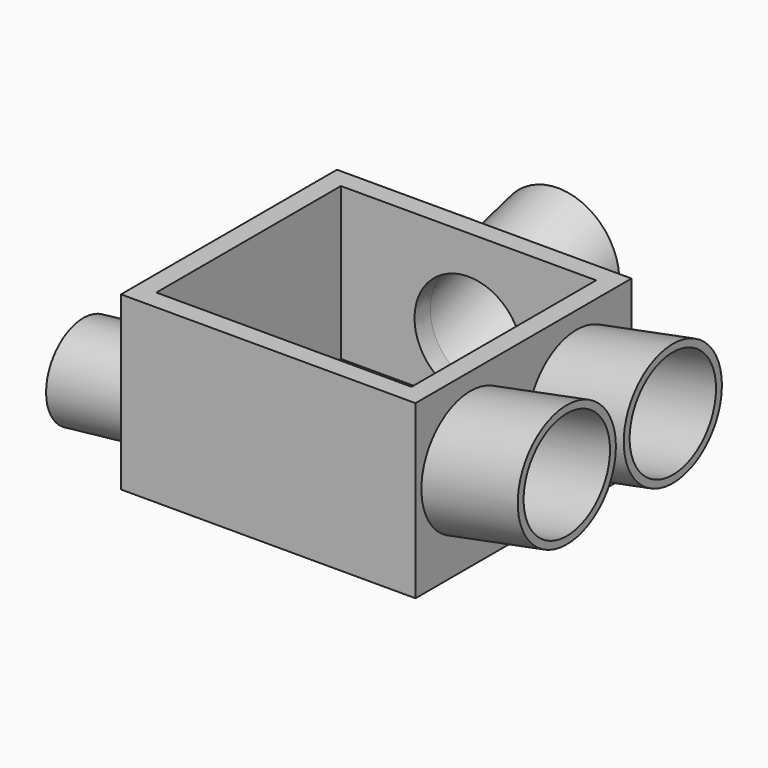
from build123d import *

# Parameters (mm, degrees)
F0_W      = 60
F0_H      = 55
F1_DEPTH  = 35
F2_T      = -4
F3_R      = 9.5
F3_R_2    = 8
F6_R      = 8
F7_DEPTH  = 4
F8_R      = 12.5
F8_R_2    = 11
F11_R     = 11
F12_DEPTH = 4
F13_R     = 12.5
F13_R_2   = 11
F16_DEPTH = 4


with BuildPart() as f1:
    # F0 (on Top) → F1 (new body)
    with BuildSketch(Plane.XY):
        Rectangle(F0_W, F0_H)
    extrude(amount=F1_DEPTH)

    # F2
    f2_openings = [f1.faces().sort_by_distance(p)[0] for p in [
        (0, 0, 35),
    ]]
    offset(amount=F2_T, openings=f2_openings)

    # F5: sweep along a path in F4
    with BuildLine(Plane.XZ) as f5_path:
        Line((-30, 12.8732416779), (-49.8803923108, 10.6892083519))
    # F3 (on face) → F5 (sweep)
    with BuildSketch(Plane(origin=(-30, 0, 0), x_dir=(0, -1, 0), z_dir=(-1, 0, 0))):
        with Locations((12.2240986817, 10.7874526048)):
            Circle(F3_R)
        with Locations((12.2240986817, 10.7874526048)):
            Circle(F3_R_2, mode=Mode.SUBTRACT)
    sweep(path=f5_path.line)

    # F6 (on face) → F7 (cut, through all)
    with BuildSketch(Plane(origin=(-30, 0, 0), x_dir=(0, -1, 0), z_dir=(-1, 0, 0))):
        with Locations((12.2240986817, 10.7874526048)):
            Circle(F6_R)
    extrude(amount=-F7_DEPTH, mode=Mode.SUBTRACT)

    # F10: sweep along a path in F9
    with BuildLine(Plane.XZ) as f10_path:
        Line((34.9448250159, 21.2307306323), (54.5700194764, 25.0845264738))
    # F8 (on face) → F10 (sweep)
    with BuildSketch(Plane.YZ.offset(30)):
        with Locations((-13.5, 19)):
            Circle(F8_R)
        with Locations((-13.5, 19)):
            Circle(F8_R_2, mode=Mode.SUBTRACT)
        with Locations((13.5, 19)):
            Circle(F8_R)
        with Locations((13.5, 19)):
            Circle(F8_R_2, mode=Mode.SUBTRACT)
    sweep(path=f10_path.line)

    # F11 (on face) → F12 (cut, through all)
    with BuildSketch(Plane.YZ.offset(30)):
        with Locations((13.5, 19)):
            Circle(F11_R)
        with Locations((-13.5, 19)):
            Circle(F11_R)
    extrude(amount=-F12_DEPTH, mode=Mode.SUBTRACT)

    # F15: sweep along a path in F14
    with BuildLine(Plane.YZ) as f15_path:
        Line((26.9883851239, 16.3239016038), (46.2833066753, 21.5875507492))
    # F13 (on face) → F15 (sweep)
    with BuildSketch(Plane(origin=(0, 27.5, 0), x_dir=(-1, 0, 0), z_dir=(0, 1, 0))):
        with Locations((0, 16.2113178521)):
            Circle(F13_R)
        with Locations((0, 16.2113178521)):
            Circle(F13_R_2, mode=Mode.SUBTRACT)
    sweep(path=f15_path.line)

    # F16 (cut, through all): a face of the model
    f16_faces = [f1.faces().sort_by_distance(p)[0] for p in [
        (5.559e-07, 27.5, 16.2113144868),
    ]]
    extrude(f16_faces, amount=-F16_DEPTH, mode=Mode.SUBTRACT)


solid = f1.part
